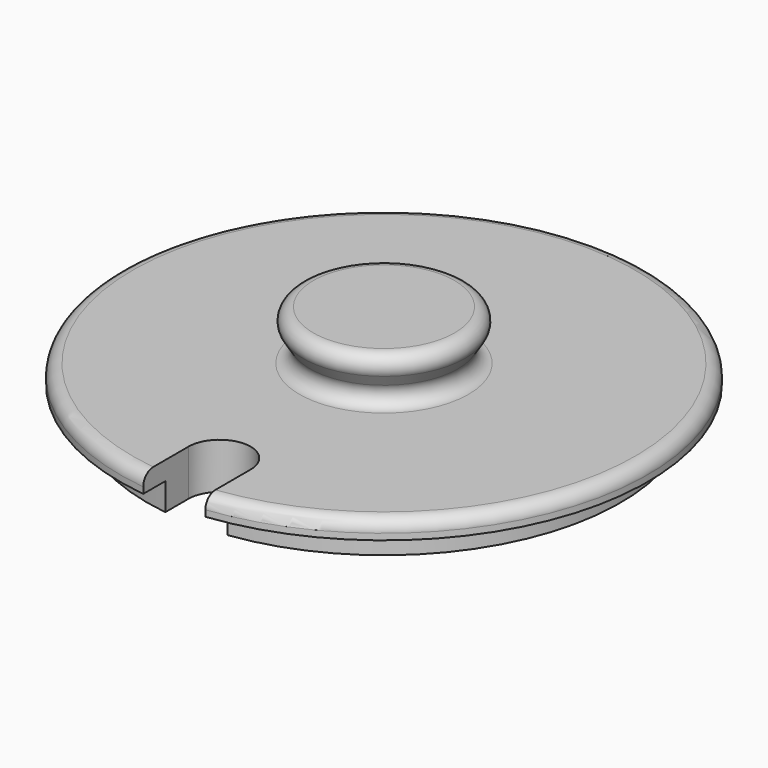
from build123d import *

# Parameters (mm, degrees)
F3_DEPTH      = 126
F3_DEPTH_BACK = 15.401


# Not quite as in the source:
# - an extrude ends at something that could not be found from the text; its depth is read off the source's solid


with BuildPart() as f1:
    # F0 (on Front) → F1 (revolve)
    with BuildSketch(Plane.XZ):
        with BuildLine():
            Line((0, 0), (38.1, 0))
            Line((38.1, 0), (38.1, 4.4))
            Line((38.1, 4.4), (42.5, 4.4))
            Line((42.5, 4.4), (42.5, 5.4))
            ThreePointArc((42.5, 5.4), (41.9142135624, 6.8142135624), (40.5, 7.4))
            Line((40.5, 7.4), (13.608495283, 7.4))
            ThreePointArc((13.608495283, 7.4), (11.8592103205, 8.4304629352), (11.912498675, 10.45999788))
            Line((11.912498675, 10.45999788), (13.087501325, 12.34000212))
            ThreePointArc((13.087501325, 12.34000212), (13.1407896795, 14.3695370648), (11.391504717, 15.4))
            Line((11.391504717, 15.4), (0, 15.4))
            Line((0, 15.4), (0, 0))
        make_face()
    revolve(axis=Axis((0, 0, 11.4377464585), (0, 0, -1)))

    # F2 (on Top) → F3 (cut, two sides)
    with BuildSketch(Plane.XY) as f3_sk:
        with BuildLine():
            ThreePointArc((5, -33.1), (0, -28.1), (-5, -33.1))
            Line((-5, -33.1), (-5, -42.5))
            Line((-5, -42.5), (5, -42.5))
            Line((5, -42.5), (5, -33.1))
        make_face()
    extrude(amount=-F3_DEPTH, mode=Mode.SUBTRACT)
    extrude(f3_sk.sketch, amount=F3_DEPTH_BACK, mode=Mode.SUBTRACT)


solid = f1.part
